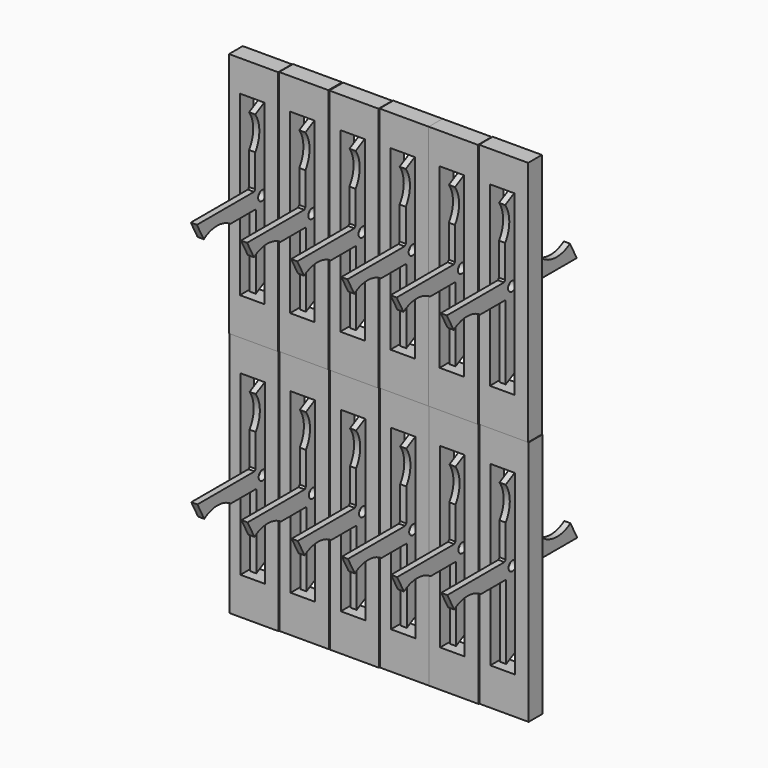
from build123d import *

# Parameters (mm, degrees)
F1_R     = 2.5
F2_DEPTH = 3.175
F0_W     = 25.4
F0_H     = 127
F0_W_2   = 12.7
F0_H_2   = 91.6145071387
F3_DEPTH = 8.89


# Not quite as in the source:
# - a feature names something its author has since deleted; it is built from what else it names
# - the program builds the solid bodies; features that only make, move or delete a surface that nothing else refers to are left out


with BuildPart() as f2:
    # F1 (on Right) → F2 (new body)
    with BuildSketch(Plane.YZ):
        with BuildLine():
            ThreePointArc((0.6285369935, 6.1646287317), (1.8144050261, 8.1246171158), (2.2276205739, 10.377857087))
            ThreePointArc((2.2276205739, 10.377857087), (1.8291751939, 12.5917896978), (0.6838418006, 14.5278857037))
            ThreePointArc((0.6838418006, 14.5278857037), (0.3003496249, 14.9343873175), (-0.1173979088, 15.3055972431))
            ThreePointArc((-0.1173979088, 15.3055972431), (-4.3572308337, 16.723512673), (-8.4806548809, 14.9960748234))
            ThreePointArc((-8.4806548809, 14.9960748234), (-8.8748564381, 14.5893250318), (-9.2312432278, 14.1490652032))
            ThreePointArc((-9.2312432278, 14.1490652032), (-10.4487815672, 9.8309238655), (-8.5082188332, 5.7858082311))
            ThreePointArc((-8.5082188332, 5.7858082311), (-8.3214546972, 5.6144269292), (-8.127999492, 5.4506359749))
            ThreePointArc((-8.127999492, 5.4506359749), (-3.8883778548, 4.0321701057), (0.2352574801, 5.7590368271))
            ThreePointArc((0.2352574801, 5.7590368271), (0.4364101194, 5.9574568925), (0.6285369935, 6.1646287317))
        make_face()
        with Locations((-4.1223794261, 10.377857087)):
            Circle(F1_R, mode=Mode.SUBTRACT)
        with BuildLine():
            ThreePointArc((0.6838418006, 14.5278857037), (1.8291751939, 12.5917896978), (2.2276205739, 10.377857087))
            ThreePointArc((2.2276205739, 10.377857087), (1.8144050261, 8.1246171158), (0.6285369935, 6.1646287317))
            Line((0.6285369935, 6.1646287317), (37.6954082937, 6.1646287317))
            Line((37.6954082937, 6.1646287317), (33.2936274446, 14.5278857037))
            ThreePointArc((33.2936274446, 14.5278857037), (24.6955792046, 11.8708569929), (16.0975309647, 14.5278857037))
            Line((16.0975309647, 14.5278857037), (0.6838418006, 14.5278857037))
        make_face()
        with BuildLine():
            ThreePointArc((-8.4806548809, 14.9960748234), (-4.3572308337, 16.723512673), (-0.1173979088, 15.3055972431))
            Line((-0.1173979088, 15.3055972431), (-0.1173979088, 53.4055972431))
            Line((-0.1173979088, 53.4055972431), (-8.4806548809, 49.003816394))
            ThreePointArc((-8.4806548809, 49.003816394), (-5.82362617, 40.405768154), (-8.4806548809, 31.8077199141))
            Line((-8.4806548809, 31.8077199141), (-8.4806548809, 14.9960748234))
        make_face()
        with BuildLine():
            Line((0.2352574801, -11.0447889214), (0.2352574801, 5.7590368271))
            ThreePointArc((0.2352574801, 5.7590368271), (-3.8883778548, 4.0321701057), (-8.127999492, 5.4506359749))
            Line((-8.127999492, 5.4506359749), (-8.127999492, -32.6426662505))
            Line((-8.127999492, -32.6426662505), (0.2352574801, -28.2408854013))
            ThreePointArc((0.2352574801, -28.2408854013), (-2.4217712308, -19.6428371614), (0.2352574801, -11.0447889214))
        make_face()
        with BuildLine():
            ThreePointArc((-8.5082188332, 5.7858082311), (-10.4487815672, 9.8309238655), (-9.2312432278, 14.1490652032))
            Line((-9.2312432278, 14.1490652032), (-46.1170420253, 14.1490652032))
            Line((-46.1170420253, 14.1490652032), (-41.7152611761, 5.7858082311))
            ThreePointArc((-41.7152611761, 5.7858082311), (-33.1172129362, 8.4428369419), (-24.5191646962, 5.7858082311))
            Line((-24.5191646962, 5.7858082311), (-8.8025887588, 5.7858082311))
            Line((-8.8025887588, 5.7858082311), (-8.5082188332, 5.7858082311))
        make_face()
    extrude(amount=F2_DEPTH)


with BuildPart() as f3:
    # F0 (on Front) → F3 (new body)
    with BuildSketch(Plane.XZ):
        with Locations((2.6480006054, 8.830661118)):
            Rectangle(F0_W, F0_H)
        with Locations((1.9292394467, 10.382976383)):
            Rectangle(F0_W_2, F0_H_2, mode=Mode.SUBTRACT)
    extrude(amount=F3_DEPTH)


with BuildPart() as f2_1:
    # F5: moved
    add(f2.part.moved(Location((-65.278, 0, 3.302))))


with BuildPart() as f3_1:
    # F5: moved
    add(f3.part.moved(Location((-65.278, 0, 3.302))))


with BuildPart() as f6_1:
    # F6: copy of F2
    add(f2_1.part.moved(Location((25.908, 0, 0.254))))


with BuildPart() as f6_2:
    # F6: copy of F3
    add(f3_1.part.moved(Location((25.908, 0, 0.254))))


with BuildPart() as f7_1:
    # F7: copy of F6_1
    add(f6_1.part.moved(Location((51.816, 0, 0.254))))


with BuildPart() as f7_2:
    # F7: copy of F6_2
    add(f6_2.part.moved(Location((51.816, 0, 0.254))))


with BuildPart() as f7_3:
    # F7: copy of F2
    add(f2_1.part.moved(Location((51.816, 0, 0.254))))


with BuildPart() as f7_4:
    # F7: copy of F3
    add(f3_1.part.moved(Location((51.816, 0, 0.254))))


with BuildPart() as f8_1:
    # F8: copy of F7_3
    add(f7_3.part.moved(Location((51.308, 0, 0.254))))


with BuildPart() as f8_2:
    # F8: copy of F7_1
    add(f7_1.part.moved(Location((51.308, 0, 0.254))))


with BuildPart() as f8_3:
    # F8: copy of F7_4
    add(f7_4.part.moved(Location((51.308, 0, 0.254))))


with BuildPart() as f8_4:
    # F8: copy of F7_2
    add(f7_2.part.moved(Location((51.308, 0, 0.254))))


with BuildPart() as f9_1:
    # F9: copy of F7_3
    add(f7_3.part.moved(Location((0.254, 0, -127))))


with BuildPart() as f9_2:
    # F9: copy of F6_1
    add(f6_1.part.moved(Location((0.254, 0, -127))))


with BuildPart() as f9_3:
    # F9: copy of F6_2
    add(f6_2.part.moved(Location((0.254, 0, -127))))


with BuildPart() as f9_4:
    # F9: copy of F8_3
    add(f8_3.part.moved(Location((0.254, 0, -127))))


with BuildPart() as f9_5:
    # F9: copy of F8_4
    add(f8_4.part.moved(Location((0.254, 0, -127))))


with BuildPart() as f9_6:
    # F9: copy of F8_2
    add(f8_2.part.moved(Location((0.254, 0, -127))))


with BuildPart() as f9_7:
    # F9: copy of F2
    add(f2_1.part.moved(Location((0.254, 0, -127))))


with BuildPart() as f9_8:
    # F9: copy of F8_1
    add(f8_1.part.moved(Location((0.254, 0, -127))))


with BuildPart() as f9_9:
    # F9: copy of F7_1
    add(f7_1.part.moved(Location((0.254, 0, -127))))


with BuildPart() as f9_10:
    # F9: copy of F3
    add(f3_1.part.moved(Location((0.254, 0, -127))))


with BuildPart() as f9_11:
    # F9: copy of F7_4
    add(f7_4.part.moved(Location((0.254, 0, -127))))


with BuildPart() as f9_12:
    # F9: copy of F7_2
    add(f7_2.part.moved(Location((0.254, 0, -127))))


solid = Compound([f2_1.part, f3_1.part, f6_1.part, f6_2.part, f7_1.part, f7_2.part, f7_3.part, f7_4.part, f8_1.part, f8_2.part, f8_3.part, f8_4.part, f9_1.part, f9_2.part, f9_3.part, f9_4.part, f9_5.part, f9_6.part, f9_7.part, f9_8.part, f9_9.part, f9_10.part, f9_11.part, f9_12.part])
